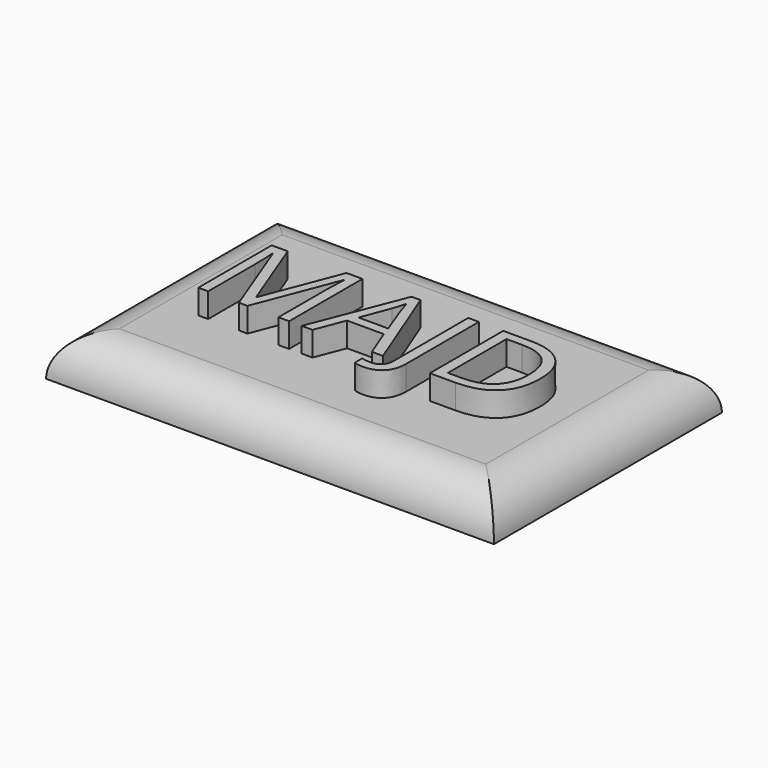
from build123d import *

# Parameters (mm, degrees)
F0_W         = 55
F0_H         = 35
F1_DEPTH     = 5
F2_R         = 4.99999
F3_TEXT_SIZE = 15.77617551
F4_DEPTH     = 3


# Not quite as in the source:
# - a fillet or chamfer is up to 0.001 mm smaller than in the source, because OpenCascade refuses the exact size
# - Text() gives the source's letters only with a copy of the font that has no kerning and outlines rounded to 1/6400 em; it was checked with that copy


with BuildPart() as f1:
    # F0 (on Top) → F1 (new body)
    with BuildSketch(Plane.XY):
        Rectangle(F0_W, F0_H)
    extrude(amount=F1_DEPTH)

    # F2 (radius 5 in the source; OpenCascade refuses exactly that, so slightly less here)
    f2_edges = [f1.edges().sort_by_distance(p)[0] for p in [
        (-27.5, 0, 5),
        (27.5, 0, 5),
        (0, -17.5, 5),
        (0, 17.5, 5),
    ]]
    fillet(f2_edges, radius=F2_R)

    # F3 (on face) → F4 (join)
    with BuildSketch(Plane.XY.offset(5)):
        with Locations((-19.8726654053, -5.6028608233)):
            Text('MAJD', F3_TEXT_SIZE, font='Open Sans', text_align=(TextAlign.LEFT, TextAlign.BOTTOM))
    extrude(amount=F4_DEPTH)


solid = f1.part
